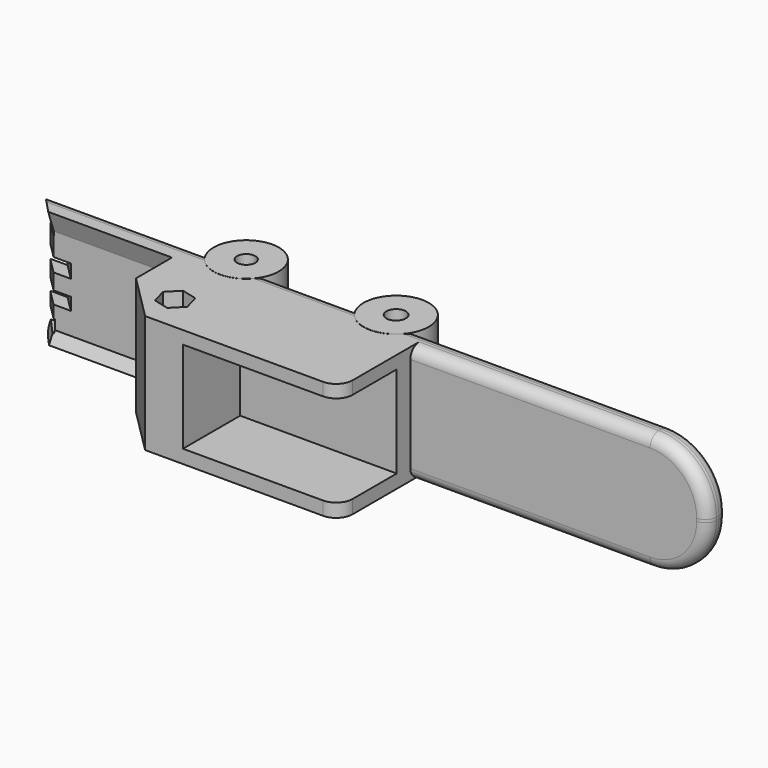
from build123d import *

# Parameters (mm, degrees)
F0_W          = 85.1304866374
F0_H          = 26.3841096312
F1_DEPTH      = 25.4
F0_W_2        = 66.4924792945
F2_DEPTH      = 5.588
F4_DEPTH      = 31.496
F5_W          = 3.8600212429
F5_H          = 3.1541939825
F5_H_2        = 3.028026782
F5_H_3        = 2.775690984
F5_W_2        = 4.1123558767
F6_DEPTH      = 25.4
F8_DEPTH      = 28.702
F9_SIZE       = 10.16
F10_R         = 3.6792614691
F11_T1_DEPTH  = 4.1635371745
F11_T3_DEPTH  = 3.532698378
F11_T5_DEPTH  = 2.7756914496
F11_T7_DEPTH  = 3.028026782
F11_T9_DEPTH  = 2.775690984
F11_T14_DEPTH = 21.9165514071
F11_T20_DEPTH = 21.7996979777
F12_R         = 12.8774151417
F13_W         = 36.6102233529
F13_H         = 20.5034988467
F14_DEPTH     = 16.002
F15_R         = 7.2867112822
F15_R_2       = 2.0440412519
F15_R_3       = 2.1726876713
F16_DEPTH     = 26.416
F17_T1_DEPTH  = 53.6150641528
F17_T3_DEPTH  = 0.6292793478
F17_T8_DEPTH  = 62.3259871722
F17_S9_R      = 7.2867112822
F17_T10_DEPTH = 33
F17_T14_DEPTH = 31.9739065533
F17_S15_R     = 7.2867112822
F17_T16_DEPTH = 18
F17_S17_R     = 7.2867112822
F17_T18_DEPTH = 18
F17_T22_DEPTH = 47.4524435023
F17_S23_R     = 7.2867112822
F17_T24_DEPTH = 25
F17_T28_DEPTH = 31.9739065533
F17_S29_R     = 7.2867112822
F17_T30_DEPTH = 18
F17_S31_R     = 7.2867112822
F17_T32_DEPTH = 18
F17_T36_DEPTH = 47.4524435023
F17_S37_R     = 7.2867112822
F17_T38_DEPTH = 25
F17_T42_DEPTH = 62.3259871722
F17_S43_R     = 7.2867112822
F17_T44_DEPTH = 33
F17_T46_ANGLE = 90
F17_T48_ANGLE = 90
F17_T50_ANGLE = 90
F17_T52_ANGLE = 90
F21_DEPTH     = 1.778
F23_DEPTH     = 1.524
F24_R         = 2.0849148325


# Not quite as in the source:
# - a fillet or chamfer that OpenCascade refuses, or shapes differently, is made with other operations: its cross-section is extruded or revolved along the edge and cut away or added


with BuildPart() as f1:
    # F0 (on Front) → F1 (new body)
    with BuildSketch(Plane.XZ):
        with Locations((42.5652433187, 13.1920548156)):
            Rectangle(F0_W, F0_H)
    extrude(amount=F1_DEPTH)

    # F0 (on Front) → F2 (join)
    with BuildSketch(Plane.XZ):
        with Locations((118.3767262846, 13.1920548156)):
            Rectangle(F0_W_2, F0_H)
    extrude(amount=F2_DEPTH)

    # F3 (on face) → F4 (cut)
    with BuildSketch(Plane(origin=(0, 0, 0), x_dir=(0, -1, 0), z_dir=(-1, 0, 0))):
        Polygon((35.6419347227, 33.0609679222), (7.6199998148, 33.5525795817), (5.1796691639, 26.3841096312), (25.4, 26.3841096312), (25.4, 0), (4.9407089369, 0), (7.8658051789, -6.022258196), (35.6419347227, -6.022258196), align=None)
        Polygon((25.4, 26.3841096312), (5.1796691639, 26.3841096312), (3.687096294, 21.9996776432), (3.687096294, 2.5809677318), (4.9407089369, 0), (25.4, 0), align=None)
    extrude(amount=-F4_DEPTH, mode=Mode.SUBTRACT)

    # F5 (on Front) → F6 (cut)
    with BuildSketch(Plane.XZ):
        with Locations((1.9300106214, 22.6104753092)):
            Rectangle(F5_W, F5_H)
        with Locations((1.9300106214, 15.3558277525)):
            Rectangle(F5_W, F5_H_2)
        with Locations((1.9300106214, 8.9212704916)):
            Rectangle(F5_W, F5_H_3)
        with Locations((2.0561779384, 3.3698880579)):
            Rectangle(F5_W_2, F5_H_3)
    extrude(amount=F6_DEPTH, mode=Mode.SUBTRACT)

    # F7 (on Top) → F8 (cut)
    with BuildSketch(Plane.XY):
        Polygon((40.8404252998, -13.7686529255), (38.3662302699, -16.301950867), (39.3230331276, -19.7113155876), (42.7540310152, -20.5873823667), (45.2282260452, -18.0540844252), (44.2714231875, -14.6447197046), align=None)
    extrude(amount=F8_DEPTH, mode=Mode.SUBTRACT)

    # F9
    f9_edges = [f1.edges().sort_by_distance(p)[0] for p in [
        (31.496, -25.4, 13.192055),
    ]]
    chamfer(f9_edges, length=F9_SIZE)

    # F10
    f10_edges = [f1.edges().sort_by_distance(p)[0] for p in [
        (85.130487, -25.4, 13.192055),
    ]]
    fillet(f10_edges, radius=F10_R)

    # F11: chamfer of 3.81 on 7 edges, made by hand

    # F11_s2 → F11_t1 (cut)
    with BuildSketch(Plane.XY.offset(16.8698411435)):
        with BuildLine():
            Line((3.9177630735, -3.7948593675), (-0.1077630735, 0.2306667794))
            Line((-0.1077630735, 0.2306667794), (-0.1839630735, 0.2306667794))
            ThreePointArc((-0.1839630735, 0.2306667794), (-0.0762, -1.7282147573), (-0.0762, -3.687096294))
            Line((-0.0762, -3.687096294), (0, -3.763296294))
            ThreePointArc((0, -3.763296294), (1.9588815367, -3.763296294), (3.9177630735, -3.8710593675))
            Line((3.9177630735, -3.8710593675), (3.9177630735, -3.7948593675))
        make_face()
    extrude(amount=F11_T1_DEPTH, mode=Mode.SUBTRACT)

    # F11_s4 → F11_t3 (cut)
    with BuildSketch(Plane.XY.offset(10.3091159835)):
        with BuildLine():
            Line((3.9177630735, -3.7948593675), (-0.1077630735, 0.2306667794))
            Line((-0.1077630735, 0.2306667794), (-0.1839630735, 0.2306667794))
            ThreePointArc((-0.1839630735, 0.2306667794), (-0.0762, -1.7282147573), (-0.0762, -3.687096294))
            Line((-0.0762, -3.687096294), (0, -3.763296294))
            ThreePointArc((0, -3.763296294), (1.9588815367, -3.763296294), (3.9177630735, -3.8710593675))
            Line((3.9177630735, -3.8710593675), (3.9177630735, -3.7948593675))
        make_face()
    extrude(amount=F11_T3_DEPTH, mode=Mode.SUBTRACT)

    # F11_s6 → F11_t5 (cut)
    with BuildSketch(Plane.XY.offset(4.7577335499)):
        with BuildLine():
            Line((3.9177630735, -3.7948593675), (-0.1077630735, 0.2306667794))
            Line((-0.1077630735, 0.2306667794), (-0.1839630735, 0.2306667794))
            ThreePointArc((-0.1839630735, 0.2306667794), (-0.0762, -1.7282147573), (-0.0762, -3.687096294))
            Line((-0.0762, -3.687096294), (0, -3.763296294))
            ThreePointArc((0, -3.763296294), (1.9588815367, -3.763296294), (3.9177630735, -3.8710593675))
            Line((3.9177630735, -3.8710593675), (3.9177630735, -3.7948593675))
        make_face()
    extrude(amount=F11_T5_DEPTH, mode=Mode.SUBTRACT)

    # F11_s8 → F11_t7 (cut)
    with BuildSketch(Plane.XY.offset(13.8418143615)):
        with BuildLine():
            Line((7.7777843163, -3.7948593675), (3.7522581694, 0.2306667794))
            Line((3.7522581694, 0.2306667794), (3.6760581694, 0.2306667794))
            ThreePointArc((3.6760581694, 0.2306667794), (3.7838212429, -1.7282147573), (3.7838212429, -3.687096294))
            Line((3.7838212429, -3.687096294), (3.8600212429, -3.763296294))
            ThreePointArc((3.8600212429, -3.763296294), (5.8189027796, -3.763296294), (7.7777843163, -3.8710593675))
            Line((7.7777843163, -3.8710593675), (7.7777843163, -3.7948593675))
        make_face()
    extrude(amount=F11_T7_DEPTH, mode=Mode.SUBTRACT)

    # F11_s10 → F11_t9 (cut)
    with BuildSketch(Plane.XY.offset(7.5334249996)):
        with BuildLine():
            Line((7.7777843163, -3.7948593675), (3.7522581694, 0.2306667794))
            Line((3.7522581694, 0.2306667794), (3.6760581694, 0.2306667794))
            ThreePointArc((3.6760581694, 0.2306667794), (3.7838212429, -1.7282147573), (3.7838212429, -3.687096294))
            Line((3.7838212429, -3.687096294), (3.8600212429, -3.763296294))
            ThreePointArc((3.8600212429, -3.763296294), (5.8189027796, -3.763296294), (7.7777843163, -3.8710593675))
            Line((7.7777843163, -3.8710593675), (7.7777843163, -3.7948593675))
        make_face()
    extrude(amount=F11_T9_DEPTH, mode=Mode.SUBTRACT)


with BuildPart() as f11_tool12:
    # F11_s13 → F11_t14 (new body)
    with BuildSketch(Plane(origin=(0, -11.7445344188, 34.4995634238), x_dir=(1, 0, 0), z_dir=(0, 0.3222638516, -0.9466498877))):
        with BuildLine():
            Line((3.9177630735, -3.491548486), (-0.1077630735, -7.5170746329))
            Line((-0.1077630735, -7.5170746329), (-0.1839630735, -7.5170746329))
            ThreePointArc((-0.1839630735, -7.5170746329), (-0.0762, -5.5581930961), (-0.0762, -3.5993115594))
            Line((-0.0762, -3.5993115594), (0, -3.5231115594))
            ThreePointArc((0, -3.5231115594), (1.9588815367, -3.5231115594), (3.9177630735, -3.415348486))
            Line((3.9177630735, -3.415348486), (3.9177630735, -3.491548486))
        make_face()
    extrude(amount=F11_T14_DEPTH)

    split(bisect_by=Plane.XY.offset(26.3841096312), keep=Keep.BOTTOM)

    split(bisect_by=Plane.XY.offset(24.1875723004), keep=Keep.TOP)


with BuildPart() as f1_1:
    add(f1.part)

    # F11_t11: cut F11_tool12
    add(f11_tool12.part, mode=Mode.SUBTRACT)


with BuildPart() as f11_tool18:
    # F11_s19 → F11_t20 (new body)
    with BuildSketch(Plane(origin=(0, 4.3004322544, 8.8538329162), x_dir=(1, 0, 0), z_dir=(0, -0.4369038907, -0.8995081936))):
        with BuildLine():
            Line((3.9177630735, 4.5519712442), (-0.1077630735, 0.5264450973))
            Line((-0.1077630735, 0.5264450973), (-0.1839630735, 0.5264450973))
            ThreePointArc((-0.1839630735, 0.5264450973), (-0.0762, 2.485326634), (-0.0762, 4.4442081707))
            Line((-0.0762, 4.4442081707), (0, 4.5204081707))
            ThreePointArc((0, 4.5204081707), (1.9588815367, 4.5204081707), (3.9177630735, 4.6281712442))
            Line((3.9177630735, 4.6281712442), (3.9177630735, 4.5519712442))
        make_face()
    extrude(amount=F11_T20_DEPTH)

    split(bisect_by=Plane.XY.offset(1.9820425659), keep=Keep.BOTTOM)


with BuildPart() as f1_2:
    add(f1_1.part)

    # F11_t17: cut F11_tool18
    add(f11_tool18.part, mode=Mode.SUBTRACT)

    # F12
    f12_edges = [f1_2.edges().sort_by_distance(p)[0] for p in [
        (151.622966, -2.794, 0),
        (151.622966, -2.794, 26.38411),
    ]]
    fillet(f12_edges, radius=F12_R)

    # F13 (on face) → F14 (cut)
    with BuildSketch(Plane.XZ.offset(25.4)):
        with Locations((68.4222616255, 13.2684203563)):
            Rectangle(F13_W, F13_H)
    extrude(amount=-F14_DEPTH, mode=Mode.SUBTRACT)

    # F15 (on face) → F16 (join)
    with BuildSketch(Plane(origin=(0, 0, 0), x_dir=(1, 0, 0), z_dir=(0, 0, -1))):
        with Locations((42.1016700566, -2.3023090325)):
            Circle(F15_R)
        with Locations((42.1016700566, -2.3023090325)):
            Circle(F15_R_2, mode=Mode.SUBTRACT)
        with Locations((75.6382346153, -2.3023090325)):
            Circle(F15_R)
        with Locations((75.6382346153, -2.3023090325)):
            Circle(F15_R_3, mode=Mode.SUBTRACT)
    extrude(amount=-F16_DEPTH)

    # F17: fillet of radius 2.4528409794 on 14 edges, made by hand

    # F17_s2 → F17_t1 (cut)
    with BuildSketch(Plane.YZ.offset(85.1304866374)):
        with BuildLine():
            ThreePointArc((-5.588, 2.4528409794), (-4.8695795103, 0.7184204897), (-3.1351590206, 0))
            Line((-3.1351590206, 0), (-5.588, 0))
            Line((-5.588, 0), (-5.588, 2.4528409794))
        make_face()
        with BuildLine():
            ThreePointArc((-3.1351590206, 26.3841096312), (-4.8695795103, 25.6656891415), (-5.588, 23.9312686518))
            Line((-5.588, 23.9312686518), (-5.588, 26.3841096312))
            Line((-5.588, 26.3841096312), (-3.1351590206, 26.3841096312))
        make_face()
    extrude(amount=F17_T1_DEPTH, mode=Mode.SUBTRACT)

    # F17_s4 → F17_t3 (cut)
    with BuildSketch(Plane.XY.offset(12.8774151417)):
        with BuildLine():
            ThreePointArc((149.1701249525, 0), (150.9045454422, -0.7184204897), (151.6229659319, -2.4528409794))
            Line((151.6229659319, -2.4528409794), (151.6229659319, 0))
            Line((151.6229659319, 0), (149.1701249525, 0))
        make_face()
        with BuildLine():
            ThreePointArc((149.1701249525, -5.588), (150.9045454422, -4.8695795103), (151.6229659319, -3.1351590206))
            Line((151.6229659319, -3.1351590206), (151.6229659319, -5.588))
            Line((151.6229659319, -5.588), (149.1701249525, -5.588))
        make_face()
    extrude(amount=F17_T3_DEPTH, mode=Mode.SUBTRACT)


with BuildPart() as f17_tool6:
    # F17_s7 → F17_t8 (new body)
    with BuildSketch(Plane.YZ.offset(76.419563618)):
        with BuildLine():
            ThreePointArc((0, 2.4528409794), (-0.7184204897, 0.7184204897), (-2.4528409794, 0))
            Line((-2.4528409794, 0), (0, 0))
            Line((0, 0), (0, 2.4528409794))
        make_face()
    extrude(amount=F17_T8_DEPTH)

    # F17_s9 → F17_t10 (cut, symmetric)
    with BuildSketch(Plane.XY.offset(1.2)):
        with Locations((75.6382346153, 2.3023090325)):
            Circle(F17_S9_R)
    extrude(amount=F17_T10_DEPTH, both=True, mode=Mode.SUBTRACT)


with BuildPart() as f1_3:
    add(f1_2.part)

    # F17_t5: cut F17_tool6
    add(f17_tool6.part, mode=Mode.SUBTRACT)


with BuildPart() as f17_tool12:
    # F17_s13 → F17_t14 (new body)
    with BuildSketch(Plane.YZ.offset(42.8829990593)):
        with BuildLine():
            ThreePointArc((0, 2.4528409794), (-0.7184204897, 0.7184204897), (-2.4528409794, 0))
            Line((-2.4528409794, 0), (0, 0))
            Line((0, 0), (0, 2.4528409794))
        make_face()
    extrude(amount=F17_T14_DEPTH)

    # F17_s15 → F17_t16 (cut, symmetric)
    with BuildSketch(Plane.XY.offset(1.2)):
        with Locations((75.6382346153, 2.3023090325)):
            Circle(F17_S15_R)
    extrude(amount=F17_T16_DEPTH, both=True, mode=Mode.SUBTRACT)

    # F17_s17 → F17_t18 (cut, symmetric)
    with BuildSketch(Plane.XY.offset(1.2)):
        with Locations((42.1016700566, 2.3023090325)):
            Circle(F17_S17_R)
    extrude(amount=F17_T18_DEPTH, both=True, mode=Mode.SUBTRACT)


with BuildPart() as f1_4:
    add(f1_3.part)

    # F17_t11: cut F17_tool12
    add(f17_tool12.part, mode=Mode.SUBTRACT)


with BuildPart() as f17_tool20:
    # F17_s21 → F17_t22 (new body)
    with BuildSketch(Plane.YZ.offset(-6.1321024484)):
        with BuildLine():
            ThreePointArc((0, 2.4528409794), (-0.7184204897, 0.7184204897), (-2.4528409794, 0))
            Line((-2.4528409794, 0), (0, 0))
            Line((0, 0), (0, 2.4528409794))
        make_face()
    extrude(amount=F17_T22_DEPTH)

    # F17_s23 → F17_t24 (cut, symmetric)
    with BuildSketch(Plane.XY.offset(1.2)):
        with Locations((42.1016700566, 2.3023090325)):
            Circle(F17_S23_R)
    extrude(amount=F17_T24_DEPTH, both=True, mode=Mode.SUBTRACT)


with BuildPart() as f1_5:
    add(f1_4.part)

    # F17_t19: cut F17_tool20
    add(f17_tool20.part, mode=Mode.SUBTRACT)


with BuildPart() as f17_tool26:
    # F17_s27 → F17_t28 (new body)
    with BuildSketch(Plane.YZ.offset(74.8569056126)):
        with BuildLine():
            ThreePointArc((-2.4528409794, 26.3841096312), (-0.7184204897, 25.6656891415), (0, 23.9312686518))
            Line((0, 23.9312686518), (0, 26.3841096312))
            Line((0, 26.3841096312), (-2.4528409794, 26.3841096312))
        make_face()
    extrude(amount=-F17_T28_DEPTH)

    # F17_s29 → F17_t30 (cut, symmetric)
    with BuildSketch(Plane.XY.offset(25.2)):
        with Locations((75.6382346153, 2.3023090325)):
            Circle(F17_S29_R)
    extrude(amount=F17_T30_DEPTH, both=True, mode=Mode.SUBTRACT)

    # F17_s31 → F17_t32 (cut, symmetric)
    with BuildSketch(Plane.XY.offset(25.2)):
        with Locations((42.1016700566, 2.3023090325)):
            Circle(F17_S31_R)
    extrude(amount=F17_T32_DEPTH, both=True, mode=Mode.SUBTRACT)


with BuildPart() as f1_6:
    add(f1_5.part)

    # F17_t25: cut F17_tool26
    add(f17_tool26.part, mode=Mode.SUBTRACT)


with BuildPart() as f17_tool34:
    # F17_s35 → F17_t36 (new body)
    with BuildSketch(Plane.YZ.offset(41.3203410539)):
        with BuildLine():
            ThreePointArc((-2.4528409794, 26.3841096312), (-0.7184204897, 25.6656891415), (0, 23.9312686518))
            Line((0, 23.9312686518), (0, 26.3841096312))
            Line((0, 26.3841096312), (-2.4528409794, 26.3841096312))
        make_face()
    extrude(amount=-F17_T36_DEPTH)

    # F17_s37 → F17_t38 (cut, symmetric)
    with BuildSketch(Plane.XY.offset(25.2)):
        with Locations((42.1016700566, 2.3023090325)):
            Circle(F17_S37_R)
    extrude(amount=F17_T38_DEPTH, both=True, mode=Mode.SUBTRACT)


with BuildPart() as f1_7:
    add(f1_6.part)

    # F17_t33: cut F17_tool34
    add(f17_tool34.part, mode=Mode.SUBTRACT)


with BuildPart() as f17_tool40:
    # F17_s41 → F17_t42 (new body)
    with BuildSketch(Plane.YZ.offset(138.7455507902)):
        with BuildLine():
            ThreePointArc((-2.4528409794, 26.3841096312), (-0.7184204897, 25.6656891415), (0, 23.9312686518))
            Line((0, 23.9312686518), (0, 26.3841096312))
            Line((0, 26.3841096312), (-2.4528409794, 26.3841096312))
        make_face()
    extrude(amount=-F17_T42_DEPTH)

    # F17_s43 → F17_t44 (cut, symmetric)
    with BuildSketch(Plane.XY.offset(25.2)):
        with Locations((75.6382346153, 2.3023090325)):
            Circle(F17_S43_R)
    extrude(amount=F17_T44_DEPTH, both=True, mode=Mode.SUBTRACT)


with BuildPart() as f1_8:
    add(f1_7.part)

    # F17_t39: cut F17_tool40
    add(f17_tool40.part, mode=Mode.SUBTRACT)

    # F17_s45 → F17_t46 (revolve, cut)
    with BuildSketch(Plane.YZ.offset(138.7455507902)):
        with BuildLine():
            ThreePointArc((-2.4528409794, 26.3841096312), (-0.7184204897, 25.6656891415), (0, 23.9312686518))
            Line((0, 23.9312686518), (0, 26.3841096312))
            Line((0, 26.3841096312), (-2.4528409794, 26.3841096312))
        make_face()
    revolve(axis=Axis((138.7455507902, 0, 13.5066944895), (0, 1, 0)), revolution_arc=F17_T46_ANGLE, mode=Mode.SUBTRACT)

    # F17_s47 → F17_t48 (revolve, cut)
    with BuildSketch(Plane.YZ.offset(138.7455507902)):
        with BuildLine():
            ThreePointArc((-3.1351590206, 26.3841096312), (-4.8695795103, 25.6656891415), (-5.588, 23.9312686518))
            Line((-5.588, 23.9312686518), (-5.588, 26.3841096312))
            Line((-5.588, 26.3841096312), (-3.1351590206, 26.3841096312))
        make_face()
    revolve(axis=Axis((138.7455507902, -5.588, 13.5066944895), (0, 1, 0)), revolution_arc=F17_T48_ANGLE, mode=Mode.SUBTRACT)

    # F17_s49 → F17_t50 (revolve, cut)
    with BuildSketch(Plane.XY.offset(12.8774151417)):
        with BuildLine():
            ThreePointArc((149.1701249525, 0), (150.9045454422, -0.7184204897), (151.6229659319, -2.4528409794))
            Line((151.6229659319, -2.4528409794), (151.6229659319, 0))
            Line((151.6229659319, 0), (149.1701249525, 0))
        make_face()
    revolve(axis=Axis((138.7455507902, 0, 12.8774151417), (0, 1, 0)), revolution_arc=F17_T50_ANGLE, mode=Mode.SUBTRACT)

    # F17_s51 → F17_t52 (revolve, cut)
    with BuildSketch(Plane.XY.offset(12.8774151417)):
        with BuildLine():
            ThreePointArc((149.1701249525, -5.588), (150.9045454422, -4.8695795103), (151.6229659319, -3.1351590206))
            Line((151.6229659319, -3.1351590206), (151.6229659319, -5.588))
            Line((151.6229659319, -5.588), (149.1701249525, -5.588))
        make_face()
    revolve(axis=Axis((138.7455507902, -5.588, 12.8774151417), (0, 1, 0)), revolution_arc=F17_T52_ANGLE, mode=Mode.SUBTRACT)

    # F20 (on offset) → F21 (join)
    with BuildSketch(Plane.XY.offset(6.096)):
        Polygon((21.6764695942, -1.2347314041), (23.9960364997, -4.4464389794), (32.8282304108, -9.7100706771), (38.6150412891, 0), (36.4860072732, 2.8691168409), align=None)
    extrude(amount=F21_DEPTH)

    # F22 (on offset) → F23 (join)
    with BuildSketch(Plane.XY.offset(18.542)):
        Polygon((21.7032115906, -1.1815896723), (24.0227784961, -4.3932972476), (32.8549724072, -9.6569289453), (38.6417832855, 0.0531417318), (36.5127492696, 2.9222585727), align=None)
    extrude(amount=-F23_DEPTH)

    # F24
    f24_edges = [f1_8.edges().sort_by_distance(p)[0] for p in [
        (31.496, -3.687096, 12.446),
        (31.496, -3.687096, 4.338484),
        (31.496, -3.687096, 20.270839),
    ]]
    fillet(f24_edges, radius=F24_R)


solid = f1_8.part
